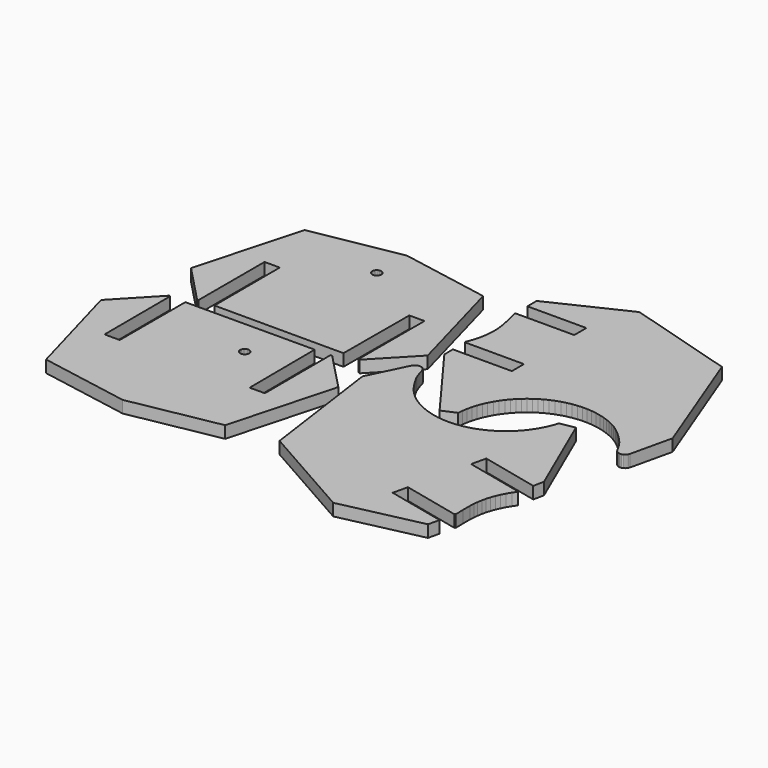
from build123d import *

# Parameters (mm, degrees)
F1_DEPTH = 6.35


with BuildPart() as f1:
    # F0 (on Top) → F1 (new body)
    with BuildSketch(Plane.XY):
        Polygon((747.5924596, -72.4337388), (737.7956542, -92.588207), (747.0914192, -158.9379346), (799.006276, -188.3485692), (841.5509712, -178.9316462), (842.920971, -172.9792578), (812.56378, -165.9923274), (814.363751, -158.171769), (843.9900062, -164.989637), (844.354928, -164.9884686), (844.6738758, -164.8111766), (844.8675, -164.5018554), (844.9076828, -164.2313708), (844.7671192, -159.700849), (844.7890394, -155.1681936), (844.908267, -152.8799584), (845.1550534, -150.6019848), (845.5285858, -148.3413086), (846.0277466, -146.1050164), (846.69884, -143.8970452), (847.498559, -141.732381), (848.4241604, -139.6184406), (849.6006376, -137.3479092), (850.9228092, -135.158988), (852.3850364, -133.061075), (852.278077, -132.7787794), (821.8214958, -125.7689636), (823.6214668, -117.9484306), (853.9942788, -124.9389424), (855.16974, -119.2865788), (835.240646, -73.2910396), (827.3978626, -74.7424972), (826.5183876, -77.342619), (825.4604268, -79.8753546), (824.2290856, -82.3284866), (822.8303076, -84.6901532), (821.2708492, -86.9489752), (819.8404736, -88.7350778), (818.3056786, -90.4323312), (816.6719506, -92.0345378), (814.945157, -93.5360334), (813.131089, -94.930722), (811.2367062, -96.2142602), (809.2688666, -97.3821014), (807.2346314, -98.429953), (804.8985426, -99.4466388), (802.500173, -100.3061748), (800.050089, -101.0048018), (797.5590856, -101.5394464), (795.0380848, -101.907721), (792.4982372, -102.1080508), (789.9506934, -102.139496), (787.4066548, -102.0019804), (784.8773482, -101.6960628), (782.5865476, -101.243511), (780.323814, -100.666804), (778.095853, -99.9677198), (775.9019026, -99.117277), (773.7627654, -98.1370402), (771.6861376, -97.0305654), (769.6691744, -95.8040502), (767.7383172, -94.445963), (765.9021512, -92.9623744), (764.1688552, -91.359863), (762.5460238, -89.6455154), (760.9645182, -87.665052), (759.4864414, -85.6062042), (757.6854798, -82.724371), (756.0355466, -79.75346), (755.1483754, -77.554074), (754.3793396, -75.3106444), (753.730649, -73.0295212), (753.4801034, -72.4101422), (753.1237414, -71.8449922), (752.672866, -71.3519528), (752.0407362, -70.9315828), (751.3284694, -70.6689214), (750.5747498, -70.5782942), (749.8205476, -70.6646034), (749.1378464, -70.905878), (748.5202962, -71.2838808), (747.9906046, -71.8057492), align=None)
    extrude(amount=F1_DEPTH)


with BuildPart() as f1b:
    # F0 (on Top) → F1, piece 2 (new body)
    with BuildSketch(Plane.XY):
        Polygon((630.4456784, -86.0316542), (610.8887452, -106.635423), (626.4143936, -162.3646994), (673.6594604, -170.8110884), (720.8478852, -162.053905), (736.006402, -106.2236636), (716.31429, -85.7490538), (715.6524676, -86.0169476), (715.795622, -129.5161494), (707.7681552, -129.5425654), (707.4788746, -86.205187), (639.2839132, -86.4296214), (639.2798746, -129.767965), (631.2523824, -129.794381), (631.109228, -86.2951792), align=None)
        Polygon((683.6652062, -105.2288726), (683.875315, -104.6101286), (684.1678722, -104.1534874), (684.551336, -103.7699982), (685.0079772, -103.477441), (685.6535182, -103.2657574), (686.3325364, -103.2448024), (686.989863, -103.4163286), (687.5721072, -103.766366), (687.9586952, -104.1485598), (688.2487886, -104.6082998), (688.4273506, -105.1217354), (688.4851356, -105.6622728), (688.429662, -106.2035214), (688.2517096, -106.7176682), (687.9606764, -107.1773828), (687.5721072, -107.558205), (687.0156186, -107.9007494), (686.386867, -108.0787272), (685.7334266, -108.0787272), (685.104675, -107.9007494), (684.5481864, -107.558205), (684.0904276, -107.0919118), (683.7769916, -106.5185322), (683.6315766, -105.8814494), align=None, mode=Mode.SUBTRACT)
    extrude(amount=F1_DEPTH)


with BuildPart() as f1c:
    # F0 (on Top) → F1, piece 3 (new body)
    with BuildSketch(Plane.XY):
        Polygon((872.3544656, -55.7767744), (848.3680772, 6.7799966), (791.1668962, 23.7553754), (751.831999, 5.0071528), (751.836444, -1.100836), (782.9872834, -1.078103), (782.9931508, -9.1031314), (752.5925258, -9.1261438), (752.3263846, -9.1853004), (752.0854148, -9.3128592), (751.8832816, -9.6653604), (751.8689814, -10.0714302), (753.043706, -14.5292572), (754.0493936, -19.0282322), (754.4396138, -21.2468714), (754.7046374, -23.483951), (754.8436516, -25.732359), (754.8561738, -27.9850342), (754.6994812, -30.2873918), (754.4073304, -32.5765414), (753.980712, -34.8444566), (753.3453056, -37.32149), (752.5495236, -39.751762), (751.5968458, -42.1249094), (751.7645874, -42.3759122), (783.0174078, -42.3530776), (783.0232752, -50.3780806), (751.8564084, -50.400839), (751.982875, -56.1727604), (781.7501764, -96.5047092), (789.0652748, -93.325823), (789.2995898, -90.7943574), (789.7015448, -88.2840754), (790.2694126, -85.806026), (791.0006532, -83.3712074), (791.8920408, -80.990313), (792.939613, -78.6739092), (794.1387724, -76.4322322), (795.4842358, -74.2751626), (796.9700088, -72.2122508), (798.4237524, -70.4451728), (799.980747, -68.7682902), (801.6353792, -67.1876228), (803.3816546, -65.7089364), (805.2133756, -64.337438), (807.1252336, -63.0796046), (809.1087196, -61.938027), (811.1566962, -60.9167692), (813.505612, -59.9261184), (815.9154624, -59.094624), (818.3754778, -58.4260198), (820.8746854, -57.9232776), (823.4018838, -57.5886326), (825.9458208, -57.4236088), (828.4950664, -57.4289428), (831.0382922, -57.6046092), (833.5640682, -57.9497952), (836.0611422, -58.4629768), (838.3345946, -59.0867246), (840.570328, -59.8344498), (842.7616114, -60.7038918), (844.8844926, -61.7363002), (846.9339424, -62.9077228), (848.900893, -64.2129526), (850.8874524, -65.7867874), (852.7908776, -67.4602664), (854.6061394, -69.2289446), (856.0568604, -70.7907652), (857.4701926, -72.3864694), (858.6511148, -74.0737152), (859.7707214, -75.8022614), (861.5734356, -78.941295), (862.0076994, -79.3913322), (862.6370098, -79.8159186), (863.347524, -80.083279), (864.100634, -80.1789354), (864.855395, -80.0976554), (865.5708622, -79.8438332), (866.1817576, -79.4551624), (866.698419, -78.947899), (867.0970974, -78.3202142), (867.3437314, -77.6187424), align=None)
    extrude(amount=F1_DEPTH)


with BuildPart() as f1d:
    # F0 (on Top) → F1, piece 4 (new body)
    with BuildSketch(Plane.XY):
        Polygon((731.8547466, -5.3739796), (684.6377468, 3.2278574), (637.420747, -5.3739796), (622.0785882, -61.1540306), (641.7032124, -81.6933342), (642.3658984, -81.4276248), (642.3658984, -37.9281944), (650.393416, -37.9281944), (650.5400756, -81.266284), (718.735418, -81.266284), (718.8820776, -37.9281944), (726.9095952, -37.9281944), (726.9095952, -81.4276248), (727.5722812, -81.6933342), (747.1969054, -61.1540306), align=None)
        Polygon((683.128936, -14.6921982), (683.5855772, -14.399641), (684.2311182, -14.1879574), (684.9101364, -14.1670024), (685.567463, -14.3385286), (686.1497072, -14.688566), (686.5362952, -15.0707598), (686.8263886, -15.5304998), (687.0049506, -16.0439354), (687.0627356, -16.5844728), (687.007262, -17.1257214), (686.8293096, -17.6398682), (686.5382764, -18.0995828), (686.1497072, -18.480405), (685.5932186, -18.8229494), (684.964467, -19.0009272), (684.3110266, -19.0009272), (683.682275, -18.8229494), (683.1257864, -18.480405), (682.6680276, -18.0141118), (682.3545916, -17.4407322), (682.2091766, -16.8036494), (682.2428062, -16.1510726), (682.452915, -15.5323286), (682.7454722, -15.0756874), align=None, mode=Mode.SUBTRACT)
    extrude(amount=F1_DEPTH)


solid = Compound([f1.part, f1b.part, f1c.part, f1d.part])
